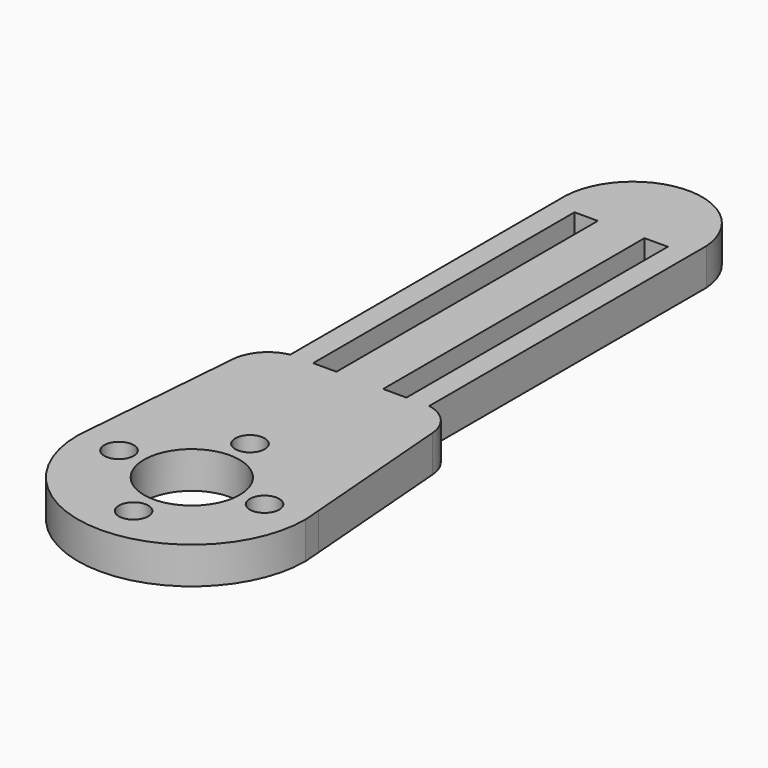
from build123d import *

# Parameters (mm, degrees)
F0_R        = 2
F0_R_2      = 6.5
F0_W        = 6.35
F0_H        = 44.45
F1_DEPTH    = 5
F2_T1_DEPTH = 28.0247734337
F2_T3_DEPTH = 27.9999173435


# Not quite as in the source:
# - a fillet or chamfer that OpenCascade refuses, or shapes differently, is made with other operations: its cross-section is extruded or revolved along the edge and cut away or added


with BuildPart() as f1:
    # F0 (on Top) → F1 (new body)
    with BuildSketch(Plane.XY):
        with BuildLine():
            Line((-13.2125969287, 28.575), (-15.3026211582, 2.4657221432))
            ThreePointArc((-15.3026211582, 2.4657221432), (0.0013716989, 15.4999999393), (15.3030573351, 2.4630136415))
            Line((15.3030573351, 2.4630136415), (13.2151419082, 28.575))
            Line((13.2151419082, 28.575), (9.4426246963, 28.575))
            Line((9.4426246963, 28.575), (9.4426246963, 75.7550326315))
            ThreePointArc((9.4426246963, 75.7550326315), (-0.1780593733, 84.4710891818), (-9.464331693, 75.3995760688))
            Line((-9.464331693, 75.3995760688), (-9.464331693, 28.575))
            Line((-9.464331693, 28.575), (-13.2125969287, 28.575))
        make_face()
        Polygon((6.35, 73.025), (6.35, 28.575), (3.175, 28.575), (-3.175, 28.575), (-6.35, 28.575), (-6.35, 73.025), (-3.175, 73.025), (3.175, 73.025), align=None, mode=Mode.SUBTRACT)
        with BuildLine():
            Line((-15.3026211582, 2.4657221432), (-15.5, 0))
            ThreePointArc((-15.5, 0), (0, -15.5), (15.5, 0))
            Line((15.5, 0), (15.3030573351, 2.4630136415))
            ThreePointArc((15.3030573351, 2.4630136415), (0.0013716989, 15.4999999393), (-15.3026211582, 2.4657221432))
        make_face()
        with Locations((-9.9, 0)):
            Circle(F0_R, mode=Mode.SUBTRACT)
        with Locations((0, -9.9)):
            Circle(F0_R, mode=Mode.SUBTRACT)
        Circle(F0_R_2, mode=Mode.SUBTRACT)
        with Locations((9.9, 0)):
            Circle(F0_R, mode=Mode.SUBTRACT)
        with Locations((0, 9.9)):
            Circle(F0_R, mode=Mode.SUBTRACT)
        with Locations((0, 50.8)):
            Rectangle(F0_W, F0_H)
    extrude(amount=F1_DEPTH)

    # F2: fillet of radius 5.08 on 2 edges, made by hand

    # F2_s2 → F2_t1 (cut)
    with BuildSketch(Plane.XY.offset(-11.5123867168)):
        with BuildLine():
            ThreePointArc((13.5821827728, 23.9846962333), (12.2908918839, 26.9818924846), (9.4426246963, 28.575))
            Line((9.4426246963, 28.575), (13.2151419082, 28.575))
            Line((13.2151419082, 28.575), (13.5821827728, 23.9846962333))
        make_face()
    extrude(amount=F2_T1_DEPTH, mode=Mode.SUBTRACT)

    # F2_s4 → F2_t3 (cut)
    with BuildSketch(Plane.XY.offset(-11.4999586717)):
        with BuildLine():
            ThreePointArc((-9.464331693, 28.575), (-12.2964780323, 26.9774445837), (-13.579647346, 23.9896840999))
            Line((-13.579647346, 23.9896840999), (-13.2125969287, 28.575))
            Line((-13.2125969287, 28.575), (-9.464331693, 28.575))
        make_face()
    extrude(amount=F2_T3_DEPTH, mode=Mode.SUBTRACT)


solid = f1.part
